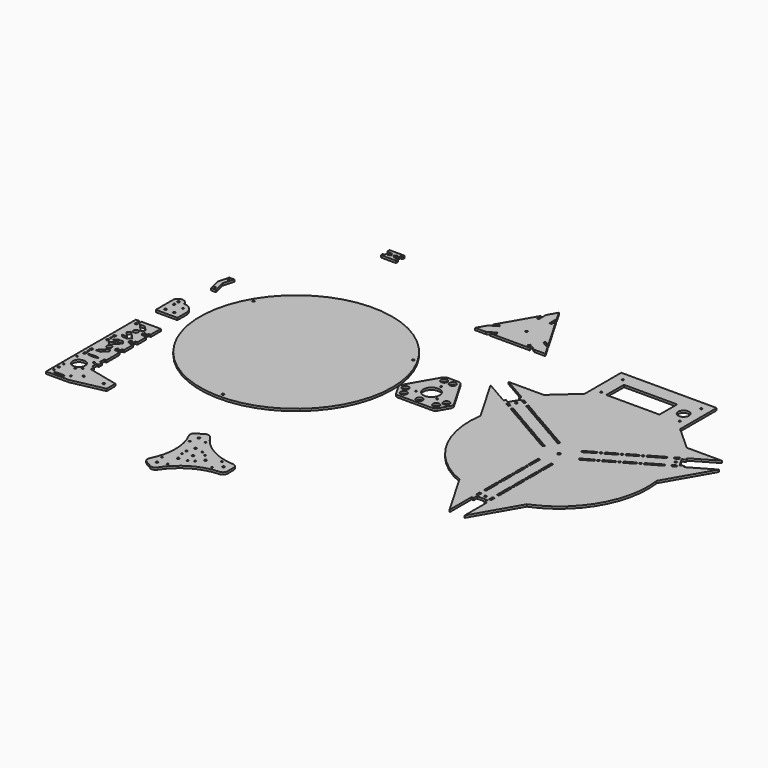
from build123d import *

# Parameters (mm, degrees)
F0_R     = 1.49999625
F0_R_2   = 1.999995
F0_R_3   = 11.4999712501
F0_W     = 3.999994
F0_H     = 4.6031024922
F0_R_4   = 4.49998875
F1_DEPTH = 4
F0_R_5   = 177.4995562511
F0_W_2   = 3.99999
F0_H_2   = 9.9561866095
F0_R_6   = 2
F0_W_3   = 19.9999510001
F0_H_3   = 3.4640928398
F0_W_4   = 3.999988
F0_H_4   = 7.9999760001
F0_R_7   = 1.9999942213
F0_W_5   = 4
F0_H_5   = 29.9999350002
F0_H_6   = 19.9999400001
F0_H_7   = 19.9999410001
F0_H_8   = 23.1915490211
F0_R_8   = 2.4999934422
F0_R_9   = 1.9999957017
F0_R_10  = 1.75
F0_R_11  = 1.9999950064
F0_R_12  = 10
F0_R_13  = 1.9999769978
F0_R_14  = 1.9999882693
F0_R_15  = 2.0033655233
F0_R_16  = 1.4940821477
F0_R_17  = 1.9930891667
F2_R     = 2
F2_R_2   = 1.5
F3_DEPTH = 4
F4_R     = 5.9
F4_R_2   = 1.5
F4_R_3   = 6
F4_R_4   = 15
F5_DEPTH = 4


# Not quite as in the source:
# - ends of sketch curves that miss each other by under 0.0002 mm in the source are joined


with BuildPart() as f1:
    # F0 (on Top) → F1 (new body)
    with BuildSketch(Plane.XY):
        Polygon((-439.5795490511, -125.5086882283), (-439.6210259474, -125.4915762711), (-440.7988980027, -125.4915762711), (-440.7988980027, -122.491583771), (-439.1989020027, -122.491583771), (-439.1989020027, -122.5621985945), (-439.1938570154, -122.5615335962), (-439.1955270112, -120.5603685991), (-435.9955370112, -120.5576966058), (-435.9938640153, -122.5615335962), (-432.9989175027, -122.5615335962), (-432.9989175027, -118.6865432836), (-428.9989275027, -118.6865432836), (-428.9989275027, -95.4949932625), (-464.8342439144, -95.4949932625), (-464.8342439144, -106.9297106757), (-468.8342339144, -106.9297106757), (-468.8342339144, -95.4949932625), (-474.998812503, -95.4949932625), (-474.998812503, -302.9560376099), (-432.9989175027, -302.9560376099), (-372.9990675023, -290.4291429271), (-372.9990675023, -270.429192927), (-428.9989275027, -257.2412538969), (-428.9989275027, -249.2412738968), (-432.9989175027, -249.2412738968), (-432.9989175027, -238.816799958), (-428.9989275027, -238.816799958), (-428.9989275027, -230.8168199579), (-432.9989175027, -230.8168199579), (-432.9989175027, -220.9362876593), (-428.9989275027, -220.9362876593), (-428.9989275027, -190.9363626591), (-432.9989175027, -190.9363626591), (-432.9989175027, -187.0613723466), (-435.9400231499, -187.0563143592), (-435.9441941395, -189.0601753496), (-439.1441871395, -189.0601753496), (-439.1400291499, -187.0664223339), (-440.7322311694, -187.0664223339), (-440.7322311694, -184.0664298339), (-439.1808460479, -184.0664298339), (-439.1425161437, -184.0613798465), (-439.1441871395, -182.0601928495), (-435.9441941395, -182.0601928495), (-435.9425231437, -184.0613798465), (-432.9989175027, -184.0613798465), (-432.9989175027, -180.186389534), (-428.9989275027, -180.186389534), (-428.9989275027, -160.1864395339), (-432.9989175027, -160.1864395339), (-432.9989175027, -156.3114492214), (-435.9656930858, -156.306413234), (-435.9640200899, -158.3102612243), (-439.16401409, -158.3102612243), (-439.1656840858, -156.3090842273), (-439.236808908, -156.2998332504), (-440.7655640861, -156.2998332504), (-440.7655640861, -153.2998407504), (-439.1681960795, -153.2998407504), (-439.1698570754, -151.3102807243), (-435.9698640753, -151.3102807243), (-435.9681930795, -153.3114567214), (-432.9989175027, -153.3114567214), (-432.9989175027, -149.4364664088), (-428.9989275027, -149.4364664088), (-428.9989275027, -129.4365164087), (-432.9989175027, -129.4365164087), (-432.9989175027, -125.5615260962), (-435.9913630216, -125.5565111087), (-435.9896930258, -127.5576771058), (-439.1896840258, -127.5603480991), (-439.1913540216, -125.559183102), align=None)
        with BuildLine():
            add(Edge.make_bspline(
                [(-445.5863090342, -297.4957282607), (-445.5863090342, -294.0828727047), (-459.7051392371, -295.7893004827), (-473.8239694401, -297.4957282607), (-459.7051392371, -299.2021560387), (-445.5863090342, -300.9085838167), (-445.5863090342, -297.4957282607)],
                knots=[0, 0, 0, 2.0943951024, 2.0943951024, 4.1887902048, 4.1887902048, 6.2831853072, 6.2831853072, 6.2831853072], degree=2, weights=[1, 0.5, 1, 0.5, 1, 0.5, 1]))
        make_face(mode=Mode.SUBTRACT)
        with Locations((-469.552397119, -291.3865105337)):
            Circle(F0_R, mode=Mode.SUBTRACT)
        with Locations((-438.4448498879, -291.3865105337)):
            Circle(F0_R, mode=Mode.SUBTRACT)
        with Locations((-469.4988262529, -280.6365374087)):
            Circle(F0_R_2, mode=Mode.SUBTRACT)
        with Locations((-469.5517851205, -268.9985985035)):
            Circle(F0_R, mode=Mode.SUBTRACT)
        with Locations((-448.2801512996, -268.9919315202)):
            Circle(F0_R, mode=Mode.SUBTRACT)
        with Locations((-423.4178604553, -280.6365374087)):
            Circle(F0_R_2, mode=Mode.SUBTRACT)
        with Locations((-386.1206556984, -280.6365374087)):
            Circle(F0_R_2, mode=Mode.SUBTRACT)
        with Locations((-453.844811388, -253.5207241982)):
            Circle(F0_R_3, mode=Mode.SUBTRACT)
        with Locations((-439.7278266804, -262.5266596833)):
            Circle(F0_R, mode=Mode.SUBTRACT)
        with Locations((-469.5258531854, -237.9090702273)):
            Circle(F0_R, mode=Mode.SUBTRACT)
        with Locations((-438.4448498879, -237.9631240922)):
            Circle(F0_R, mode=Mode.SUBTRACT)
        with Locations((-467.4761833095, -222.8868237829)):
            Rectangle(F0_W, F0_H, mode=Mode.SUBTRACT)
        with BuildLine():
            add(Edge.make_bspline(
                [(-442.6737393156, -222.7585111037), (-442.6737393156, -219.3456555477), (-456.7925695186, -221.0520833257), (-470.9113997215, -222.7585111037), (-456.7925695186, -224.4649388817), (-442.6737393156, -226.1713666597), (-442.6737393156, -222.7585111037)],
                knots=[0, 0, 0, 2.0943951024, 2.0943951024, 4.1887902048, 4.1887902048, 6.2831853072, 6.2831853072, 6.2831853072], degree=2, weights=[1, 0.5, 1, 0.5, 1, 0.5, 1]))
        make_face(mode=Mode.SUBTRACT)
        with Locations((-467.4988312529, -214.9663525841)):
            Circle(F0_R, mode=Mode.SUBTRACT)
        Polygon((-469.4761793095, -205.1884330289), (-465.4761863095, -205.1884330289), (-465.4761863095, -209.8352954118), (-469.4761803095, -209.8352954118), align=None, mode=Mode.SUBTRACT)
        Polygon((-451.9988700028, -205.9363251592), (-461.4988462529, -205.9363251592), (-452.1737155657, -195.9363501591), (-451.9988700028, -195.9363501591), (-451.9814170465, -195.7301356747), (-447.2921947695, -190.7015612461), (-442.4988937528, -195.9363501591), align=None, mode=Mode.SUBTRACT)
        with Locations((-451.9988700028, -185.5664260839)):
            Circle(F0_R_4, mode=Mode.SUBTRACT)
        Polygon((-465.5654720863, -167.7282536794), (-465.5654720863, -172.3313561716), (-469.5654650863, -172.3313561716), (-469.5654660863, -167.7282536794), align=None, mode=Mode.SUBTRACT)
        with Locations((-467.5654690863, -162.2343414141)):
            Circle(F0_R, mode=Mode.SUBTRACT)
        Polygon((-456.7275011812, -180.397214007), (-461.4988462529, -175.186402034), (-451.9988700028, -165.1864270339), (-461.4988462529, -165.1864270339), (-456.7488581278, -159.9989750026), (-447.3363046592, -159.9989750026), (-442.6737393156, -165.1864270339), align=None, mode=Mode.SUBTRACT)
        Polygon((-469.5654650863, -152.3314141715), (-465.5654720863, -152.3314141715), (-465.5654720863, -156.9782765543), (-469.5654660863, -156.9782765543), align=None, mode=Mode.SUBTRACT)
        Polygon((-456.7055452361, -129.2017149957), (-442.4988937528, -144.4364789088), (-447.2488818778, -149.62400094), (-456.7488581278, -149.62400094), (-461.4988462529, -144.4364789088), (-451.9988700028, -144.4364789088), (-461.4988462529, -134.4365039087), align=None, mode=Mode.SUBTRACT)
        with Locations((-451.9988700028, -123.991580021)):
            Circle(F0_R_4, mode=Mode.SUBTRACT)
        Polygon((-451.8240234399, -103.6865807835), (-442.4988937528, -113.6865557836), (-447.2921947695, -118.9213456966), (-461.4988462529, -103.6865807835), align=None, mode=Mode.SUBTRACT)
    extrude(amount=F1_DEPTH)


with BuildPart() as f1b:
    # F0 (on Top) → F1, piece 2 (new body)
    with BuildSketch(Plane.XY):
        with Locations((-231.1251601871, -29.9759380602)):
            Circle(F0_R_5)
        with Locations((-231.1251601871, -199.2255149362)):
            Circle(F0_R_2, mode=Mode.SUBTRACT)
        with Locations((-378.5313116717, 55.8541043647)):
            Circle(F0_R_2, mode=Mode.SUBTRACT)
        with Locations((-83.6997907505, 56.0153949615)):
            Circle(F0_R_2, mode=Mode.SUBTRACT)
    extrude(amount=F1_DEPTH)


with BuildPart() as f1c:
    # F0 (on Top) → F1, piece 3 (new body)
    with BuildSketch(Plane.XY):
        Polygon((-442.7478361304, 91.5328801678), (-451.8370994072, 91.5328801678), (-457.283592791, 71.5697730756), (-451.8370994072, 49.5329861675), (-442.7478361304, 49.5329861493), (-448.1943295142, 71.5697720756), align=None)
        with Locations((-448.8326909183, 54.9859315352)):
            Circle(F0_R, mode=Mode.SUBTRACT)
        with Locations((-448.7918990202, 86.0799338002)):
            Circle(F0_R, mode=Mode.SUBTRACT)
    extrude(amount=F1_DEPTH)


with BuildPart() as f1d:
    # F0 (on Top) → F1, piece 4 (new body)
    with BuildSketch(Plane.XY):
        Polygon((-312.8262449344, 291.4364354089), (-314.8593918515, 291.4364354089), (-314.8610558474, 289.4432753918), (-318.0610468474, 289.4459463851), (-318.0593768516, 291.4471123822), (-321.0518233704, 291.4420963948), (-321.0518233704, 287.5671060822), (-324.999187502, 287.5671060822), (-324.999187502, 282.9560946098), (-296.999187502, 282.9560946098), (-296.999187502, 287.5671060822), (-300.9465516336, 287.5671060822), (-300.9465516336, 291.4420963948), (-303.9389981525, 291.4471123822), (-303.9373281567, 289.4459463851), (-303.9431711421, 289.4459415081), (-303.9431711421, 289.4432753918), (-307.1373191567, 289.4432753918), (-307.1373191567, 296.4432597708), (-307.1373191567, 296.4459268852), (-303.9431711421, 296.4459268852), (-303.9414991462, 294.4420888948), (-303.9389981525, 294.4420888948), (-300.9465516336, 294.4420888948), (-300.9465516336, 298.3170792073), (-296.999187502, 298.3170792073), (-296.999187502, 302.9560946098), (-324.999187502, 302.9560946098), (-324.999187502, 298.3171372072), (-321.0518233704, 298.3170792073), (-321.0518233704, 294.4420888948), (-318.0568758578, 294.4420888948), (-318.055203862, 296.4459268852), (-314.855212862, 296.4432548919), (-314.8568828578, 294.4420888948), (-314.8139219652, 294.4364279089), (-312.8262449344, 294.4364279089), align=None)
        Polygon((-307.1414921463, 294.4420888948), (-307.1414921463, 291.4364354089), (-309.1721300697, 291.4364354089), (-309.1721300697, 294.4364279089), (-309.1721300697, 294.4420888948), align=None, mode=Mode.SUBTRACT)
    extrude(amount=F1_DEPTH)


with BuildPart() as f1e:
    # F0 (on Top) → F1, piece 5 (new body)
    with BuildSketch(Plane.XY):
        Polygon((-1.8421003947, 285.6355719111), (-11.8420763948, 302.9560366099), (-21.8420513949, 285.6355719111), (-21.8420513949, 272.2152924618), (-1.8421003947, 272.2152924618), align=None)
        Polygon((16.4874262814, 195.434410914), (18.4874214067, 198.8985040612), (9.8651113372, 203.8765973085), (7.8651163372, 200.4125039687), align=None)
        Polygon((28.4873965199, 216.2189689089), (30.4873917815, 219.6830622923), (21.8650813373, 224.6611553471), (19.8650863373, 221.1970620073), align=None)
        with Locations((0.1578946053, 263.7731063172)):
            Rectangle(F0_W_2, F0_H_2)
        Polygon((-1.8421003947, 258.7950130125), (-1.8421003947, 268.751199622), (-21.8420513949, 268.751199622), (-21.8420513949, 258.7950130125), (-25.8420413949, 258.7950130125), (-25.8420413949, 268.751199622), (-25.8420413949, 272.2152924618), (-25.8420413949, 278.7073862315), (-62.7938540154, 214.7049692376), (-57.1715370057, 217.9510153453), (-54.1715435711, 219.6830622923), (-45.5492331269, 224.6611553471), (-43.5492381269, 221.1970630073), (-52.1715487116, 216.2189696768), (-42.1715730107, 198.8985041684), (-33.5492631268, 203.8765973085), (-31.5492681268, 200.4125049687), (-40.1715780711, 195.434411414), (-43.1715704387, 193.7023648085), (-48.7938880153, 190.4563178592), (25.1097362257, 190.4563178592), (19.4874189347, 193.7023643176), (16.4874262814, 195.434410914), (7.8651163372, 200.4125039687), (9.8651113372, 203.8765973085), (18.4874214067, 198.8985040612), (28.4873965199, 216.2189689089), (19.8650863373, 221.1970620073), (21.8650813373, 224.6611553471), (30.4873917815, 219.6830622923), (33.4873845882, 217.9510157079), (39.1097022257, 214.7049692376), (2.1578896053, 278.7073862315), (2.1578896053, 272.2152924618), (2.1578896053, 268.751199622), (2.1578896053, 258.7950130125), align=None)
        with Locations((-11.8420758948, 227.9562243465)):
            Circle(F0_R_6, mode=Mode.SUBTRACT)
        with Locations((-23.8420463949, 263.7731063172)):
            Rectangle(F0_W_2, F0_H_2)
        Polygon((-45.1715655711, 197.1664575839), (-55.1715419814, 214.4869227571), (-66.7938440154, 207.776783558), (-76.7938190155, 190.4563178592), (-56.7938680153, 190.4563178592), align=None)
        Polygon((-45.5492331269, 224.6611553471), (-54.1715435711, 219.6830622923), (-52.1715487116, 216.2189696768), (-43.5492381269, 221.1970630073), align=None)
        Polygon((-33.5492631268, 203.8765973085), (-42.1715730107, 198.8985041684), (-40.1715780711, 195.434411414), (-31.5492681268, 200.4125049687), align=None)
        Polygon((43.1096922258, 207.776782558), (31.4873892815, 214.4869222827), (21.4874140575, 197.1664574245), (33.1097162257, 190.4563178592), (53.1096672258, 190.4563178592), align=None)
        Polygon((21.4874140575, 197.1664574245), (31.4873892815, 214.4869222827), (28.4873965199, 216.2189689089), (18.4874214067, 198.8985040612), align=None)
        with Locations((-11.8420758948, 270.4832460419)):
            Rectangle(F0_W_3, F0_H_3)
        Polygon((-52.1715487116, 216.2189696768), (-55.1715419814, 214.4869227571), (-45.1715655711, 197.1664575839), (-42.1715730107, 198.8985041684), align=None)
    extrude(amount=F1_DEPTH)


with BuildPart() as f1f:
    # F0 (on Top) → F1, piece 6 (new body)
    with BuildSketch(Plane.XY):
        with BuildLine():
            Line((131.7235082388, 88.5993365017), (66.7513821215, 88.5993365017))
            Line((66.7513821215, 88.5993365017), (111.0197374507, 63.0409903975))
            Line((111.0197374507, 63.0409903975), (109.0197424506, 59.5768970578))
            Line((109.0197424506, 59.5768970578), (115.1252134995, 56.0519168039))
            Line((115.1252134995, 56.0519168039), (105.1252384995, 38.7314511051))
            Line((105.1252384995, 38.7314511051), (99.0197737631, 42.2564432926))
            Line((99.0197737631, 42.2564432926), (97.0197787631, 38.7923499528))
            Line((97.0197787631, 38.7923499528), (52.7514171215, 64.3506861233))
            Line((52.7514171215, 64.3506861233), (100.9852385369, -19.1927430181))
            ThreePointArc((100.9852385369, -19.1927430181), (121.3444904617, -123.6659645283), (201.6413278967, -193.5342051645))
            Line((201.6413278967, -193.5342051645), (249.8751493121, -277.0776343059))
            Line((249.8751493121, -277.0776343059), (249.8751493121, -225.9609400976))
            Line((249.8751493121, -225.9609400976), (253.8751393121, -225.9609400976))
            Line((253.8751393121, -225.9609400976), (253.8751393121, -218.9109567226))
            Line((253.8751393121, -218.9109567226), (273.8750893123, -218.9109567226))
            Line((273.8750893123, -218.9109567226), (273.8750893123, -225.9609400976))
            Line((273.8750893123, -225.9609400976), (277.8750793123, -225.9609400976))
            Line((277.8750793123, -225.9609400976), (277.8750793123, -277.0776343059))
            Line((277.8750793123, -277.0776343059), (326.1089007277, -193.5342051645))
            ThreePointArc((326.1089007277, -193.5342051645), (406.4100868046, -123.6684751011), (426.7649910875, -19.1927430181))
            Line((426.7649910875, -19.1927430181), (474.998812503, 64.3506861233))
            Line((474.998812503, 64.3506861233), (430.7304571739, 38.7923390192))
            Line((430.7304571739, 38.7923390192), (428.7304621738, 42.2564323589))
            Line((428.7304621738, 42.2564323589), (422.6249974375, 38.7314401714))
            Line((422.6249974375, 38.7314401714), (412.6250224374, 56.0519058702))
            Line((412.6250224374, 56.0519058702), (418.7304871738, 59.5768970578))
            Line((418.7304871738, 59.5768970578), (416.7304921738, 63.0409903975))
            Line((416.7304921738, 63.0409903975), (460.9988465029, 88.5993365017))
            Line((460.9988465029, 88.5993365017), (396.0267213856, 88.5993365017))
            Line((396.0267213856, 88.5993365017), (352.1159646784, 128.1467825174))
            Line((352.1159646784, 128.1467825174), (352.1159646784, 212.6197069883))
            Line((352.1159646784, 212.6197069883), (175.634264946, 212.6197069883))
            Line((175.634264946, 212.6197069883), (175.634264946, 128.1467825174))
            Line((175.634264946, 128.1467825174), (131.7235082388, 88.5993365017))
        make_face()
        with Locations((251.8751113122, -211.5364981588)):
            Rectangle(F0_W_4, F0_H_4, mode=Mode.SUBTRACT)
        with Locations((263.8751143122, -211.5364761588)):
            Circle(F0_R_7, mode=Mode.SUBTRACT)
        with Locations((275.8750793123, -211.5364771588)):
            Rectangle(F0_W_4, F0_H_4, mode=Mode.SUBTRACT)
        with Locations((251.8751443121, -182.65599636)):
            Rectangle(F0_W_5, F0_H_5, mode=Mode.SUBTRACT)
        with Locations((275.8750793123, -182.65599636)):
            Rectangle(F0_W_4, F0_H_5, mode=Mode.SUBTRACT)
        with Locations((251.8751443121, -162.2810432974)):
            Circle(F0_R_6, mode=Mode.SUBTRACT)
        with Locations((275.8750793123, -162.2810432974)):
            Circle(F0_R_6, mode=Mode.SUBTRACT)
        with Locations((206.4286084064, -22.0654858745)):
            Circle(F0_R_6, mode=Mode.SUBTRACT)
        Polygon((210.0834857913, -26.4850257874), (212.0834807913, -23.0209324477), (232.1679543738, -34.6167053514), (230.1679575801, -38.080800798), align=None, mode=Mode.SUBTRACT)
        Polygon((183.4532703668, -11.1100642248), (185.4532653668, -7.6459708851), (202.7737310657, -17.6459458851), (200.7737360657, -21.1100392249), align=None, mode=Mode.SUBTRACT)
        with Locations((179.798393129, -6.6905240572)):
            Circle(F0_R_6, mode=Mode.SUBTRACT)
        Polygon((222.0834571602, -5.7004653779), (224.0834521603, -2.2363720381), (244.1679225802, -13.8321504196), (242.1679275802, -17.2962427594), align=None, mode=Mode.SUBTRACT)
        with Locations((218.4285798248, -1.2809253793)):
            Circle(F0_R_6, mode=Mode.SUBTRACT)
        with Locations((251.8751443121, -146.9060877348)):
            Rectangle(F0_W_5, F0_H_6, mode=Mode.SUBTRACT)
        with Locations((275.8750793123, -146.9060877348)):
            Rectangle(F0_W_4, F0_H_6, mode=Mode.SUBTRACT)
        with Locations((251.8751443121, -131.5311201722)):
            Circle(F0_R_6, mode=Mode.SUBTRACT)
        with Locations((251.8751443121, -116.1561521096)):
            Rectangle(F0_W_5, F0_H_7, mode=Mode.SUBTRACT)
        with Locations((275.8750793123, -131.5311201722)):
            Circle(F0_R_6, mode=Mode.SUBTRACT)
        with Locations((275.8750793123, -116.1561521096)):
            Rectangle(F0_W_4, F0_H_7, mode=Mode.SUBTRACT)
        with Locations((251.8751443121, -100.781196047)):
            Circle(F0_R_6, mode=Mode.SUBTRACT)
        with Locations((275.8750793123, -100.781196047)):
            Circle(F0_R_6, mode=Mode.SUBTRACT)
        with Locations((251.8751443121, -83.8104359739)):
            Rectangle(F0_W_5, F0_H_8, mode=Mode.SUBTRACT)
        with Locations((275.8750793123, -83.8104359739)):
            Rectangle(F0_W_4, F0_H_8, mode=Mode.SUBTRACT)
        with Locations((263.8751148122, -41.3758700603)):
            Circle(F0_R_8, mode=Mode.SUBTRACT)
        Polygon((283.5823070442, -13.8321504196), (303.666778833, -2.2363754091), (305.6667738331, -5.7004677488), (285.5823020442, -17.2962427594), align=None, mode=Mode.SUBTRACT)
        Polygon((295.5822770443, -34.6167084582), (315.6667488331, -23.0209324477), (317.6667438331, -26.4850257874), (297.5822720443, -38.080800798), align=None, mode=Mode.SUBTRACT)
        with Locations((321.3216211994, -22.0654858423)):
            Circle(F0_R_6, mode=Mode.SUBTRACT)
        with Locations((309.3216511993, -1.2809283037)):
            Circle(F0_R_6, mode=Mode.SUBTRACT)
        Polygon((326.9764935588, -21.1100392249), (324.9764985587, -17.6459458851), (342.2969632576, -7.6459708851), (344.2969582576, -11.1100642248), align=None, mode=Mode.SUBTRACT)
        with Locations((347.9518356204, -6.6905242737)):
            Circle(F0_R_6, mode=Mode.SUBTRACT)
        Polygon((114.9758125605, 33.0442053895), (112.9758175605, 29.5801120497), (106.0476318809, 33.5801020497), (108.0476268809, 37.0441953895), align=None, mode=Mode.SUBTRACT)
        with Locations((116.5117067207, 43.7044327389)):
            Circle(F0_R_9, mode=Mode.SUBTRACT)
        Polygon((123.5326041685, 28.1039387402), (149.5133012167, 13.1039772401), (147.5133062167, 9.6398839003), (121.5326091685, 24.6398464004), align=None, mode=Mode.SUBTRACT)
        with Locations((153.1681786016, 8.6844373271)):
            Circle(F0_R_6, mode=Mode.SUBTRACT)
        Polygon((176.1435156412, -2.2709843225), (174.1435206412, -5.7350776623), (156.8230559424, 4.2648973378), (158.8230509424, 7.7289906775), align=None, mode=Mode.SUBTRACT)
        with Locations((165.1681505852, 29.4689988013)):
            Circle(F0_R_6, mode=Mode.SUBTRACT)
        Polygon((197.4532363669, 13.1385871535), (214.7737010657, 3.1386121535), (212.7737075016, -0.3254786258), (195.4532413669, 9.6744938138), align=None, mode=Mode.SUBTRACT)
        with Locations((191.79836558, 14.0940364945)):
            Circle(F0_R_6, mode=Mode.SUBTRACT)
        Polygon((170.8230209424, 28.5135487161), (188.1434866413, 18.5135737161), (186.1434933597, 15.0494834263), (168.8230259424, 25.0494553764), align=None, mode=Mode.SUBTRACT)
        Polygon((135.5325741686, 48.8884967788), (161.5132712168, 33.8885352787), (159.5132782179, 30.4244454784), (133.5325791686, 45.424404439), align=None, mode=Mode.SUBTRACT)
        Polygon((118.047601881, 54.3646600883), (120.047596881, 57.8287534281), (126.9757873939, 53.8287717997), (124.9757875605, 50.3646700883), align=None, mode=Mode.SUBTRACT)
        with Locations((191.1711761168, 146.9972811108)):
            Circle(F0_R_10, mode=Mode.SUBTRACT)
        Polygon((314.9765235587, -0.3254811863), (312.9765285587, 3.1386111535), (330.2969932575, 13.1385861535), (332.2969882575, 9.6744938138), align=None, mode=Mode.SUBTRACT)
        with Locations((335.9518656203, 14.0940332649)):
            Circle(F0_R_6, mode=Mode.SUBTRACT)
        Polygon((341.6067379832, 15.0494803763), (339.6067429831, 18.5135727161), (356.927207682, 28.5135477161), (358.927202682, 25.0494553764), align=None, mode=Mode.SUBTRACT)
        Polygon((353.6067079832, -5.7350776623), (351.6067129832, -2.2709843225), (368.9271776821, 7.7289906775), (370.9271726821, 4.2648973378), align=None, mode=Mode.SUBTRACT)
        with Locations((374.5820500414, 8.6844372949)):
            Circle(F0_R_6, mode=Mode.SUBTRACT)
        Polygon((378.2369274077, 13.1039772401), (404.2176244559, 28.1039387402), (406.2176194559, 24.6398464004), (380.2369224077, 9.6398839003), align=None, mode=Mode.SUBTRACT)
        with Locations((362.5820800413, 29.4689948335)):
            Circle(F0_R_6, mode=Mode.SUBTRACT)
        Polygon((419.7026027435, 37.0441953895), (421.7025977435, 33.5801020497), (414.774412064, 29.5801120497), (412.774417064, 33.0442053895), align=None, mode=Mode.SUBTRACT)
        Polygon((368.2369524076, 30.4244419389), (366.2369574076, 33.8885342787), (392.2176518071, 48.8885013665), (394.2176494559, 45.424404439), align=None, mode=Mode.SUBTRACT)
        with Locations((411.2385224037, 43.7044327389)):
            Circle(F0_R_11, mode=Mode.SUBTRACT)
        Polygon((402.7744420639, 50.3646700883), (400.7744470639, 53.8287634281), (407.7026327434, 57.8287534281), (409.7026277434, 54.3646600883), align=None, mode=Mode.SUBTRACT)
        with Locations((336.3553861168, 146.9972811108)):
            Circle(F0_R_10, mode=Mode.SUBTRACT)
        with Locations((191.3553861168, 196.9446491108)):
            Circle(F0_R_10, mode=Mode.SUBTRACT)
        Polygon((300.6485231095, 185.6192490275), (300.350809158, 144.8960076725), (202.150809158, 144.8960076725), (202.4485231095, 185.6192490275), align=None, mode=Mode.SUBTRACT)
        with Locations((326.0473194219, 168.8628891764)):
            Circle(F0_R_12, mode=Mode.SUBTRACT)
        with Locations((336.3553861168, 196.9972811108)):
            Circle(F0_R_10, mode=Mode.SUBTRACT)
    extrude(amount=F1_DEPTH)


with BuildPart() as f1g:
    # F0 (on Top) → F1, piece 7 (new body)
    with BuildSketch(Plane.XY):
        with BuildLine():
            Line((-431.8410253974, -53.4667563331), (-431.8410253974, -33.466806333))
            ThreePointArc((-431.8410253974, -33.466806333), (-437.6988751291, -19.3247060645), (-451.8409753976, -13.4668563329))
            ThreePointArc((-451.8409753976, -13.4668563329), (-461.7902973253, -4.6085405914), (-471.8277604306, -13.3668565829))
            Line((-471.8277604306, -13.3668565829), (-471.8409253977, -13.4668563329))
            Line((-471.8409253977, -13.4668563329), (-471.8409253977, -53.4667563331))
            Line((-471.8409253977, -53.4667563331), (-431.8410253974, -53.4667563331))
        make_face()
        with Locations((-461.840950873, -43.4667625831)):
            Circle(F0_R_13, mode=Mode.SUBTRACT)
        with Locations((-445.8659251778, -43.4667725675)):
            Circle(F0_R_14, mode=Mode.SUBTRACT)
        with Locations((-461.840950873, -23.4747163132)):
            Circle(F0_R_15, mode=Mode.SUBTRACT)
        with Locations((-443.8431728921, -25.5569271077)):
            Circle(F0_R_16, mode=Mode.SUBTRACT)
        with Locations((-461.840950873, -13.4589708526)):
            Circle(F0_R_17, mode=Mode.SUBTRACT)
    extrude(amount=F1_DEPTH)


with BuildPart() as f3:
    # F2 (on Top) → F3 (new body)
    with BuildSketch(Plane.XY):
        with BuildLine():
            Line((-173.3191576007, -312.3464409502), (-185.7394526007, -319.5173019502))
            ThreePointArc((-185.7394526007, -319.5173019502), (-189.5272888895, -324.3374721499), (-188.9380147581, -330.4394800316))
            ThreePointArc((-188.9380147581, -330.4394800316), (-177.8813236007, -375.8740039502), (-188.9380148359, -421.3085278286))
            ThreePointArc((-188.9380148359, -421.3085278286), (-189.5272888895, -427.4105357506), (-185.7394525664, -432.2307058908))
            Line((-185.7394525664, -432.2307058908), (-173.3191576007, -439.4015669502))
            ThreePointArc((-173.3191576007, -439.4015669502), (-167.2508489819, -440.2718443354), (-162.2609918166, -436.7105138119))
            ThreePointArc((-162.2609918166, -436.7105138119), (-128.4418856195, -404.4178770248), (-83.566088559, -391.2759908533))
            ThreePointArc((-83.566088559, -391.2759908533), (-77.9869574035, -388.7353126425), (-75.7064856007, -383.0448649502))
            Line((-75.7064856007, -383.0448649502), (-75.7064856007, -368.7031429502))
            ThreePointArc((-75.7064856007, -368.7031429502), (-77.9869574035, -363.012695258), (-83.5660885958, -360.4720178441))
            ThreePointArc((-83.5660885958, -360.4720178441), (-128.4418856195, -347.3301308757), (-162.2609917909, -315.0374940721))
            ThreePointArc((-162.2609917909, -315.0374940721), (-167.2508489819, -311.476163565), (-173.3191576007, -312.3464409502))
        make_face()
        with Locations((-172.9373796007, -424.3985879502)):
            Circle(F2_R, mode=Mode.SUBTRACT)
        with Locations((-156.9805416007, -419.5396239502)):
            Circle(F2_R_2, mode=Mode.SUBTRACT)
        with Locations((-176.9547986007, -408.0074809502)):
            Circle(F2_R_2, mode=Mode.SUBTRACT)
        with Locations((-161.4547986007, -381.1606929502)):
            Circle(F2_R_2, mode=Mode.SUBTRACT)
        with Locations((-156.4575676007, -395.8547149502)):
            Circle(F2_R, mode=Mode.SUBTRACT)
        with Locations((-141.4805416007, -392.6928359502)):
            Circle(F2_R_2, mode=Mode.SUBTRACT)
        with Locations((-144.9216986007, -375.8740039502)):
            Circle(F2_R, mode=Mode.SUBTRACT)
        with Locations((-132.0091126007, -387.3950559502)):
            Circle(F2_R_2, mode=Mode.SUBTRACT)
        with Locations((-121.8499606007, -375.8740039502)):
            Circle(F2_R, mode=Mode.SUBTRACT)
        with Locations((-101.0091126007, -387.3950559502)):
            Circle(F2_R_2, mode=Mode.SUBTRACT)
        with Locations((-88.8903356007, -375.8740039502)):
            Circle(F2_R, mode=Mode.SUBTRACT)
        with Locations((-161.3317336007, -370.5705259502)):
            Circle(F2_R_2, mode=Mode.SUBTRACT)
        with Locations((-176.8317336007, -343.7237389502)):
            Circle(F2_R_2, mode=Mode.SUBTRACT)
        with Locations((-156.4575676007, -355.8932929502)):
            Circle(F2_R, mode=Mode.SUBTRACT)
        with Locations((-141.3574766007, -359.0383839502)):
            Circle(F2_R_2, mode=Mode.SUBTRACT)
        with Locations((-172.9373796007, -327.3494199502)):
            Circle(F2_R, mode=Mode.SUBTRACT)
        with Locations((-156.8574766007, -332.1915959502)):
            Circle(F2_R_2, mode=Mode.SUBTRACT)
        with Locations((-132.0091126007, -364.3307699502)):
            Circle(F2_R_2, mode=Mode.SUBTRACT)
        with Locations((-101.0091126007, -364.3307699502)):
            Circle(F2_R_2, mode=Mode.SUBTRACT)
    extrude(amount=F3_DEPTH)


with BuildPart() as f5:
    # F4 (on Top) → F5 (new body)
    with BuildSketch(Plane.XY):
        with BuildLine():
            ThreePointArc((-48.2087481727, -14.7499999003), (-49.280545, -18.75), (-48.2087481727, -22.7500000997))
            Line((-48.2087481727, -22.7500000997), (-38.393793, -39.75))
            ThreePointArc((-38.393793, -39.75), (-35.4655899501, -42.6782032591), (-31.46559, -43.75))
            Line((-31.46559, -43.75), (31.465589, -43.75))
            ThreePointArc((31.465589, -43.75), (35.4655891667, -42.6782031341), (38.3937924227, -39.7499996667))
            Line((38.3937924227, -39.7499996667), (48.208747, -22.75))
            ThreePointArc((48.208747, -22.75), (49.280544, -18.75), (48.2087471727, -14.7499999003))
            Line((48.2087471727, -14.7499999003), (16.743157, 39.75))
            ThreePointArc((16.743157, 39.75), (13.8149539501, 42.6782032591), (9.814954, 43.75))
            Line((9.814954, 43.75), (-9.814955, 43.75))
            ThreePointArc((-9.814955, 43.75), (-13.8149549501, 42.6782032591), (-16.7431581727, 39.7500000997))
            Line((-16.7431581727, 39.7500000997), (-48.2087481727, -14.7499999003))
        make_face()
        with Locations((-30, -32.707513)):
            Circle(F4_R, mode=Mode.SUBTRACT)
        with Locations((-37.912879, -19.002006)):
            Circle(F4_R, mode=Mode.SUBTRACT)
        with Locations((-19.485572, -17.5)):
            Circle(F4_R_2, mode=Mode.SUBTRACT)
        with Locations((0, -34.25)):
            Circle(F4_R_3, mode=Mode.SUBTRACT)
        with Locations((30, -32.707513)):
            Circle(F4_R, mode=Mode.SUBTRACT)
        with Locations((19.485571, -17.5)):
            Circle(F4_R_2, mode=Mode.SUBTRACT)
        with Locations((0, -6.25)):
            Circle(F4_R_4, mode=Mode.SUBTRACT)
        with Locations((37.912878, -19.002006)):
            Circle(F4_R, mode=Mode.SUBTRACT)
        with Locations((-7.912879, 32.959519)):
            Circle(F4_R, mode=Mode.SUBTRACT)
        with Locations((0, 16.25)):
            Circle(F4_R_2, mode=Mode.SUBTRACT)
        with Locations((7.912878, 32.959519)):
            Circle(F4_R, mode=Mode.SUBTRACT)
    extrude(amount=F5_DEPTH)


solid = Compound([f1.part, f1b.part, f1c.part, f1d.part, f1e.part, f1f.part, f1g.part, f3.part, f5.part])
